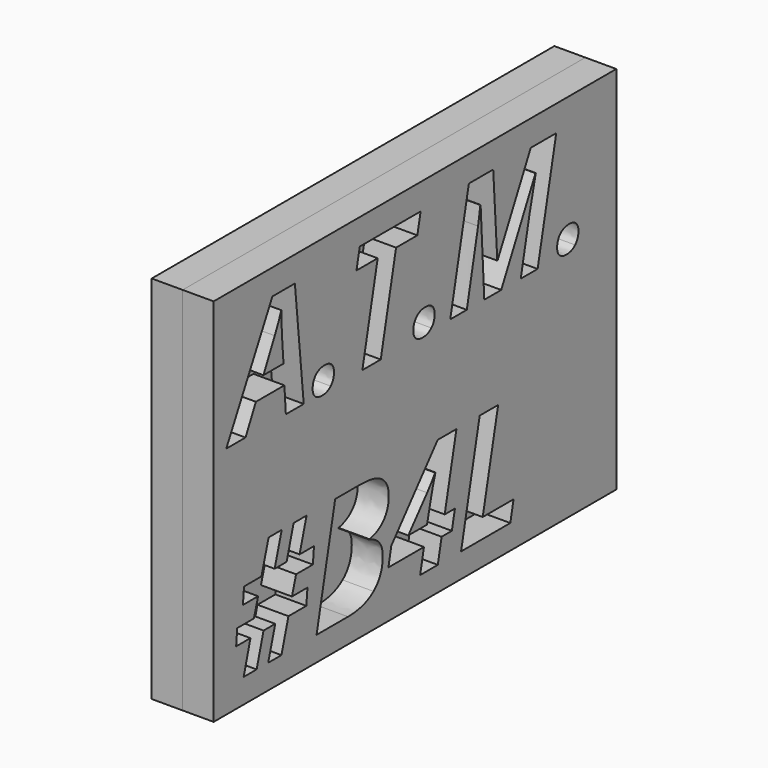
from build123d import *

# Parameters (mm, degrees)
F0_W     = 103.1923890114
F0_H     = 75.9069211781
F1_DEPTH = 6.35
F2_DEPTH = 3.81
F3_W     = 103.1923890114
F3_H     = 75.9069211781
F4_DEPTH = 6.35


with BuildPart() as f1:
    # F0 (on Right) → F1 (new body)
    with BuildSketch(Plane.YZ):
        with Locations((-0.1025758684, -4.6159606427)):
            Rectangle(F0_W, F0_H)
        Polygon((-26.2638321559, -24.5110770629), (-30.5681896813, -24.5110770629), (-31.6356308128, -28.0939234532), (-27.6524939982, -28.0939234532), (-27.9440635665, -31.2764794192), (-32.5301069461, -31.2764794192), (-34.3240010698, -37.5773472091), (-37.7190568906, -37.5773472091), (-35.9152790528, -31.2764794192), (-38.9100444493, -31.2764794192), (-40.6841711447, -37.5773472091), (-44.0050991092, -37.5773472091), (-42.2606235564, -31.2764794192), (-45.9373652314, -31.2764794192), (-45.6606212344, -28.0939234532), (-41.3809729944, -28.0939234532), (-40.2987062917, -24.5110770629), (-44.1928896786, -24.5110770629), (-43.9112038245, -21.2840443831), (-39.4487068722, -21.2840443831), (-37.6103360347, -14.9980021646), (-34.2597569276, -14.9980021646), (-36.0684766226, -21.2840443831), (-32.9946415125, -21.2840443831), (-31.2056892459, -14.9980021646), (-27.8847612814, -14.9980021646), (-29.673713548, -21.2840443831), (-25.9821463017, -21.2840443831), align=None, mode=Mode.SUBTRACT)
        with BuildLine():
            Line((-20.5510453598, -14.9980021646), (-13.9684917158, -14.9980021646))
            add(Edge.make_bspline(
                [(-13.9684917158, -14.9980021646), (-10.4350638964, -14.9980021646), (-8.62881513, -16.2581757225)],
                knots=[0, 0, 0, 1, 1, 1], degree=2))
            add(Edge.make_bspline(
                [(-8.62881513, -16.2581757225), (-6.8225663636, -17.5183492805), (-6.8225663636, -20.0189289681)],
                knots=[0, 0, 0, 1, 1, 1], degree=2))
            add(Edge.make_bspline(
                [(-6.8225663636, -20.0189289681), (-6.8225663636, -22.3366599433), (-8.1025073499, -23.8414554272)],
                knots=[0, 0, 0, 1, 1, 1], degree=2))
            add(Edge.make_bspline(
                [(-8.1025073499, -23.8414554272), (-9.3824483362, -25.3462509111), (-11.7446560253, -25.8404366202)],
                knots=[0, 0, 0, 1, 1, 1], degree=2))
            Line((-11.7446560253, -25.8404366202), (-11.7446560253, -25.9343319049))
            add(Edge.make_bspline(
                [(-11.7446560253, -25.9343319049), (-10.2027966132, -26.3346223292), (-9.2836111944, -27.4243018175)],
                knots=[0, 0, 0, 1, 1, 1], degree=2))
            add(Edge.make_bspline(
                [(-9.2836111944, -27.4243018175), (-8.3644257757, -28.5139813059), (-8.3644257757, -30.2090382878)],
                knots=[0, 0, 0, 1, 1, 1], degree=2))
            add(Edge.make_bspline(
                [(-8.3644257757, -30.2090382878), (-8.3644257757, -33.7474079643), (-10.7266334647, -35.6623775867)],
                knots=[0, 0, 0, 1, 1, 1], degree=2))
            add(Edge.make_bspline(
                [(-10.7266334647, -35.6623775867), (-13.0888411538, -37.5773472091), (-17.2597685378, -37.5773472091)],
                knots=[0, 0, 0, 1, 1, 1], degree=2))
            Line((-17.2597685378, -37.5773472091), (-25.3199374517, -37.5773472091))
            Line((-25.3199374517, -37.5773472091), (-20.5510453598, -14.9980021646))
        make_face(mode=Mode.SUBTRACT)
        Polygon((10.1378871695, -29.1910157272), (9.3521318922, -32.8974085448), (6.7230639203, -32.8974085448), (5.7495180736, -37.5773472091), (1.2277188362, -37.5773472091), (2.2012646829, -32.8974085448), (-6.9115197912, -32.8974085448), (-6.1702412277, -29.2849110119), (5.719866931, -14.9980021646), (10.5233520226, -14.9980021646), (7.5137610547, -29.1910157272), align=None, mode=Mode.SUBTRACT)
        Polygon((24.3309007322, -37.5773472091), (11.7143395813, -37.5773472091), (16.4832316732, -14.9980021646), (21.2125889084, -14.9980021646), (17.2591032363, -33.623861537), (25.1660745804, -33.623861537), align=None, mode=Mode.SUBTRACT)
        with BuildLine():
            add(Edge.make_bspline(
                [(-25.6905767334, 5.5996581868), (-26.3231344409, 6.1778554664), (-26.3231344409, 7.2107035982)],
                knots=[0, 0, 0, 1, 1, 1], degree=2))
            add(Edge.make_bspline(
                [(-26.3231344409, 7.2107035982), (-26.3231344409, 8.6043072976), (-25.4953733784, 9.4370102173)],
                knots=[0, 0, 0, 1, 1, 1], degree=2))
            add(Edge.make_bspline(
                [(-25.4953733784, 9.4370102173), (-24.6676123158, 10.2697131369), (-23.1702296175, 10.2697131369)],
                knots=[0, 0, 0, 1, 1, 1], degree=2))
            add(Edge.make_bspline(
                [(-23.1702296175, 10.2697131369), (-22.1225559144, 10.2697131369), (-21.4899982069, 9.6841030718)],
                knots=[0, 0, 0, 1, 1, 1], degree=2))
            add(Edge.make_bspline(
                [(-21.4899982069, 9.6841030718), (-20.8574404993, 9.0984930066), (-20.8574404993, 8.0310518752)],
                knots=[0, 0, 0, 1, 1, 1], degree=2))
            add(Edge.make_bspline(
                [(-20.8574404993, 8.0310518752), (-20.8574404993, 6.6868667467), (-21.7049689903, 5.854163827)],
                knots=[0, 0, 0, 1, 1, 1], degree=2))
            add(Edge.make_bspline(
                [(-21.7049689903, 5.854163827), (-22.5524974812, 5.0214609073), (-23.9263337523, 5.0214609073)],
                knots=[0, 0, 0, 1, 1, 1], degree=2))
            add(Edge.make_bspline(
                [(-23.9263337523, 5.0214609073), (-25.0580190259, 5.0214609073), (-25.6905767334, 5.5996581868)],
                knots=[0, 0, 0, 1, 1, 1], degree=2))
        make_face(mode=Mode.SUBTRACT)
        Polygon((-33.1972576532, 5.4365769029), (-33.567896935, 10.8133174169), (-40.8719617141, 10.8133174169), (-43.5257389715, 5.4365769029), (-48.4675960615, 5.4365769029), (-36.641732045, 28.1098172321), (-30.879526678, 28.1098172321), (-28.6112142736, 5.4365769029), align=None, mode=Mode.SUBTRACT)
        Polygon((-4.9496025264, 24.0327851328), (-8.8734370559, 5.4365769029), (-13.5830268628, 5.4365769029), (-9.6591923333, 24.0327851328), (-15.0952351323, 24.0327851328), (-14.2452357128, 28.0159219474), (1.3512652634, 28.0159219474), (0.5012658439, 24.0327851328), align=None, mode=Mode.SUBTRACT)
        with BuildLine():
            add(Edge.make_bspline(
                [(0.1158009909, 5.5996581868), (-0.5167567166, 6.1778554664), (-0.5167567166, 7.2107035982)],
                knots=[0, 0, 0, 1, 1, 1], degree=2))
            add(Edge.make_bspline(
                [(-0.5167567166, 7.2107035982), (-0.5167567166, 8.6043072976), (0.311004346, 9.4370102173)],
                knots=[0, 0, 0, 1, 1, 1], degree=2))
            add(Edge.make_bspline(
                [(0.311004346, 9.4370102173), (1.1387654085, 10.2697131369), (2.6361481068, 10.2697131369)],
                knots=[0, 0, 0, 1, 1, 1], degree=2))
            add(Edge.make_bspline(
                [(2.6361481068, 10.2697131369), (3.6838218099, 10.2697131369), (4.3163795175, 9.6841030718)],
                knots=[0, 0, 0, 1, 1, 1], degree=2))
            add(Edge.make_bspline(
                [(4.3163795175, 9.6841030718), (4.948937225, 9.0984930066), (4.948937225, 8.0310518752)],
                knots=[0, 0, 0, 1, 1, 1], degree=2))
            add(Edge.make_bspline(
                [(4.948937225, 8.0310518752), (4.948937225, 6.6868667467), (4.101408734, 5.854163827)],
                knots=[0, 0, 0, 1, 1, 1], degree=2))
            add(Edge.make_bspline(
                [(4.101408734, 5.854163827), (3.2538802431, 5.0214609073), (1.8800439721, 5.0214609073)],
                knots=[0, 0, 0, 1, 1, 1], degree=2))
            add(Edge.make_bspline(
                [(1.8800439721, 5.0214609073), (0.7483586984, 5.0214609073), (0.1158009909, 5.5996581868)],
                knots=[0, 0, 0, 1, 1, 1], degree=2))
        make_face(mode=Mode.SUBTRACT)
        with BuildLine():
            add(Edge.make_bspline(
                [(36.9622874544, 5.5996581868), (36.3297297469, 6.1778554664), (36.3297297469, 7.2107035982)],
                knots=[0, 0, 0, 1, 1, 1], degree=2))
            add(Edge.make_bspline(
                [(36.3297297469, 7.2107035982), (36.3297297469, 8.6043072976), (37.1574908095, 9.4370102173)],
                knots=[0, 0, 0, 1, 1, 1], degree=2))
            add(Edge.make_bspline(
                [(37.1574908095, 9.4370102173), (37.9852518721, 10.2697131369), (39.4826345704, 10.2697131369)],
                knots=[0, 0, 0, 1, 1, 1], degree=2))
            add(Edge.make_bspline(
                [(39.4826345704, 10.2697131369), (40.5303082734, 10.2697131369), (41.162865981, 9.6841030718)],
                knots=[0, 0, 0, 1, 1, 1], degree=2))
            add(Edge.make_bspline(
                [(41.162865981, 9.6841030718), (41.7954236885, 9.0984930066), (41.7954236885, 8.0310518752)],
                knots=[0, 0, 0, 1, 1, 1], degree=2))
            add(Edge.make_bspline(
                [(41.7954236885, 8.0310518752), (41.7954236885, 6.6868667467), (40.9478951976, 5.854163827)],
                knots=[0, 0, 0, 1, 1, 1], degree=2))
            add(Edge.make_bspline(
                [(40.9478951976, 5.854163827), (40.1003667066, 5.0214609073), (38.7265304356, 5.0214609073)],
                knots=[0, 0, 0, 1, 1, 1], degree=2))
            add(Edge.make_bspline(
                [(38.7265304356, 5.0214609073), (37.5948451619, 5.0214609073), (36.9622874544, 5.5996581868)],
                knots=[0, 0, 0, 1, 1, 1], degree=2))
        make_face(mode=Mode.SUBTRACT)
        with BuildLine():
            Line((20.9951471964, 11.1345381277), (21.0593913386, 11.1345381277))
            Line((21.0593913386, 11.1345381277), (29.5692692477, 28.0159219474))
            Line((29.5692692477, 28.0159219474), (36.1024043207, 28.0159219474))
            Line((36.1024043207, 28.0159219474), (31.3285703717, 5.4365769029))
            Line((31.3285703717, 5.4365769029), (27.0044454179, 5.4365769029))
            Line((27.0044454179, 5.4365769029), (29.2431066797, 16.1258137887))
            add(Edge.make_bspline(
                [(29.2431066797, 16.1258137887), (30.0634549567, 19.9359856051), (30.8640358053, 22.9356928588)],
                knots=[0, 0, 0, 1, 1, 1], degree=2))
            Line((30.8640358053, 22.9356928588), (30.7899079489, 22.9356928588))
            Line((30.7899079489, 22.9356928588), (21.9983441857, 5.4365769029))
            Line((21.9983441857, 5.4365769029), (17.6593936606, 5.4365769029))
            Line((17.6593936606, 5.4365769029), (16.7204408135, 22.9356928588))
            Line((16.7204408135, 22.9356928588), (16.6561966713, 22.9356928588))
            add(Edge.make_bspline(
                [(16.6561966713, 22.9356928588), (16.4881735303, 21.576682159), (16.0705866062, 19.3676720398)],
                knots=[0, 0, 0, 1, 1, 1], degree=2))
            add(Edge.make_bspline(
                [(16.0705866062, 19.3676720398), (15.6529996821, 17.1586619205), (13.182071137, 5.4365769029)],
                knots=[0, 0, 0, 1, 1, 1], degree=2))
            Line((13.182071137, 5.4365769029), (8.9370158967, 5.4365769029))
            Line((8.9370158967, 5.4365769029), (13.7059079886, 28.0159219474))
            Line((13.7059079886, 28.0159219474), (19.9474734933, 28.0159219474))
            Line((19.9474734933, 28.0159219474), (20.9951471964, 11.1345381277))
        make_face(mode=Mode.SUBTRACT)
    extrude(amount=F1_DEPTH)


with BuildPart() as f1b:
    # F0 (on Right) → F1, piece 2 (new body)
    with BuildSketch(Plane.YZ):
        with BuildLine():
            Line((-38.9396955919, 14.826105374), (-33.8001642182, 14.826105374))
            Line((-33.8001642182, 14.826105374), (-34.2004546425, 20.2324970305))
            add(Edge.make_bspline(
                [(-34.2004546425, 20.2324970305), (-34.3536522123, 22.2537165804), (-34.3536522123, 24.1365641317)],
                knots=[0, 0, 0, 1, 1, 1], degree=2))
            Line((-34.3536522123, 24.1365641317), (-34.3536522123, 24.6949939828))
            add(Edge.make_bspline(
                [(-34.3536522123, 24.6949939828), (-35.0356284907, 22.8417975741), (-36.03882548, 20.7711594533)],
                knots=[0, 0, 0, 1, 1, 1], degree=2))
            Line((-36.03882548, 20.7711594533), (-38.9396955919, 14.826105374))
        make_face()
    extrude(amount=F1_DEPTH)


with BuildPart() as f1c:
    # F0 (on Right) → F1, piece 3 (new body)
    with BuildSketch(Plane.YZ):
        with BuildLine():
            Line((-1.8164651313, -29.1910157272), (2.9870199602, -29.1910157272))
            Line((2.9870199602, -29.1910157272), (3.8814960935, -25.3610764824))
            add(Edge.make_bspline(
                [(3.8814960935, -25.3610764824), (4.0692866629, -24.4666003491), (4.5016991583, -22.8283747238)],
                knots=[0, 0, 0, 1, 1, 1], degree=2))
            add(Edge.make_bspline(
                [(4.5016991583, -22.8283747238), (4.9341116537, -21.1901490984), (5.1515533657, -20.6514866756)],
                knots=[0, 0, 0, 1, 1, 1], degree=2))
            Line((5.1515533657, -20.6514866756), (5.057658081, -20.6514866756))
            add(Edge.make_bspline(
                [(5.057658081, -20.6514866756), (4.5140538011, -21.6250325223), (3.0166711028, -23.4485777886)],
                knots=[0, 0, 0, 1, 1, 1], degree=2))
            Line((3.0166711028, -23.4485777886), (-1.8164651313, -29.1910157272))
        make_face()
    extrude(amount=F1_DEPTH)


with BuildPart() as f2:
    # F0 (on Right) → F2 (new body)
    with BuildSketch(Plane.YZ):
        with BuildLine():
            Line((-16.6568619728, -18.9218366941), (-17.7243031042, -23.9427634976))
            Line((-17.7243031042, -23.9427634976), (-15.4213977003, -23.9427634976))
            add(Edge.make_bspline(
                [(-15.4213977003, -23.9427634976), (-13.5533757202, -23.9427634976), (-12.6193647302, -23.1916012199)],
                knots=[0, 0, 0, 1, 1, 1], degree=2))
            add(Edge.make_bspline(
                [(-12.6193647302, -23.1916012199), (-11.6853537402, -22.4404389422), (-11.6853537402, -21.0369515286)],
                knots=[0, 0, 0, 1, 1, 1], degree=2))
            add(Edge.make_bspline(
                [(-11.6853537402, -21.0369515286), (-11.6853537402, -18.9218366941), (-14.309479855, -18.9218366941)],
                knots=[0, 0, 0, 1, 1, 1], degree=2))
            Line((-14.309479855, -18.9218366941), (-16.6568619728, -18.9218366941))
        make_face()
    extrude(amount=-F2_DEPTH)


with BuildPart() as f2b:
    # F0 (on Right) → F2, piece 2 (new body)
    with BuildSketch(Plane.YZ):
        with BuildLine():
            Line((-18.5100583816, -27.7381097427), (-19.7751737966, -33.623861537))
            Line((-19.7751737966, -33.623861537), (-16.997850112, -33.623861537))
            add(Edge.make_bspline(
                [(-16.997850112, -33.623861537), (-15.189130417, -33.623861537), (-14.1636950708, -32.7269144752)],
                knots=[0, 0, 0, 1, 1, 1], degree=2))
            add(Edge.make_bspline(
                [(-14.1636950708, -32.7269144752), (-13.1382597247, -31.8299674133), (-13.1382597247, -30.2436312874)],
                knots=[0, 0, 0, 1, 1, 1], degree=2))
            add(Edge.make_bspline(
                [(-13.1382597247, -30.2436312874), (-13.1382597247, -27.7381097427), (-15.9650019802, -27.7381097427)],
                knots=[0, 0, 0, 1, 1, 1], degree=2))
            Line((-15.9650019802, -27.7381097427), (-18.5100583816, -27.7381097427))
        make_face()
    extrude(amount=-F2_DEPTH)


with BuildPart() as f4:
    # F3 (on face) → F4 (new body)
    with BuildSketch(Plane(origin=(0, 0, 0), x_dir=(0, -1, 0), z_dir=(-1, 0, 0))):
        with Locations((0.1025758684, -4.6159606427)):
            Rectangle(F3_W, F3_H)
    extrude(amount=F4_DEPTH)


solid = Compound([f1.part, f1b.part, f1c.part, f2.part, f2b.part, f4.part])
